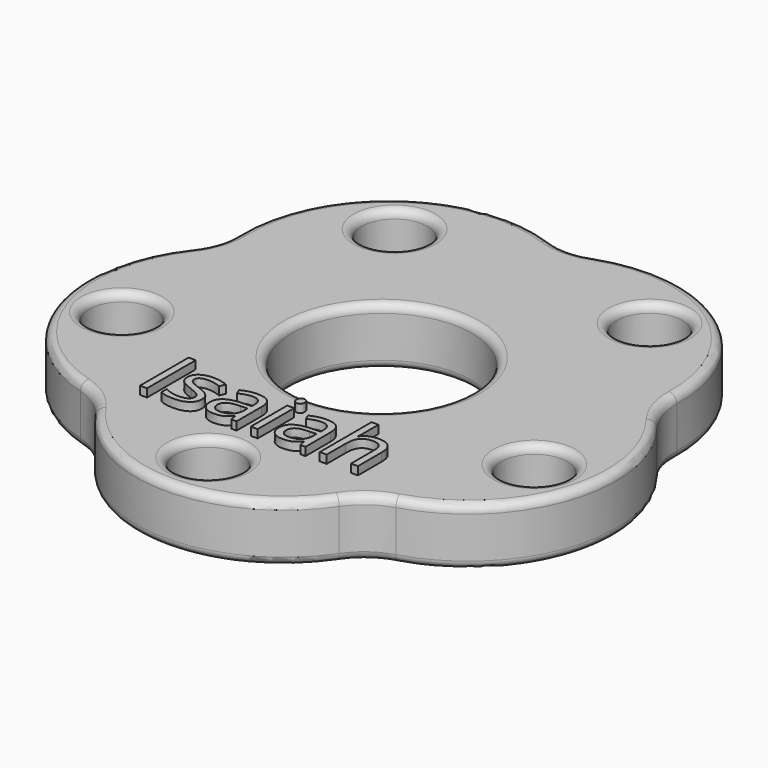
from build123d import *

# Parameters (mm, degrees)
F0_R           = 4
F0_R_2         = 11
F1_DEPTH       = 7.05
F2_R           = 8
F3_R           = 1
F4_TEXT_SIZE   = 10.4166666667
F5_DEPTH       = 1
F6_TEXT_SIZE   = 5.5555555556
F6_TEXT_SIZE_2 = 6.9444444444
F7_DEPTH       = 0.5


# Not quite as in the source:
# - Text() gives the source's letters only with a copy of the font that has no kerning and outlines rounded to 1/6400 em; it was checked with that copy


with BuildPart() as f1:
    # F0 (on Top) → F1 (new body)
    with BuildSketch(Plane.XY):
        with BuildLine():
            ThreePointArc((26.4660662972, 8.5993462218), (19.3969133257, 26.6975608144), (0, 27.8280689357))
            ThreePointArc((0, 27.8280689357), (-19.3969133257, 26.6975608144), (-26.4660662972, 8.5993462218))
            ThreePointArc((-26.4660662972, 8.5993462218), (-31.3848650377, -10.1975608144), (-16.3569285202, -22.5133806896))
            ThreePointArc((-16.3569285202, -22.5133806896), (0, -33), (16.3569285202, -22.5133806896))
            ThreePointArc((16.3569285202, -22.5133806896), (31.3848650377, -10.1975608144), (26.4660662972, 8.5993462218))
        make_face()
        with Locations((0, -26.5)):
            Circle(F0_R, mode=Mode.SUBTRACT)
        with Locations((-25.2029976818, -8.1889503509)):
            Circle(F0_R, mode=Mode.SUBTRACT)
        with Locations((25.2029976818, -8.1889503509)):
            Circle(F0_R, mode=Mode.SUBTRACT)
        Circle(F0_R_2, mode=Mode.SUBTRACT)
        with Locations((-15.5763091858, 21.4389503509)):
            Circle(F0_R, mode=Mode.SUBTRACT)
        with Locations((15.5763091858, 21.4389503509)):
            Circle(F0_R, mode=Mode.SUBTRACT)
    extrude(amount=F1_DEPTH)

    # F2
    f2_edges = [f1.edges().sort_by_distance(p)[0] for p in [
        (16.356929, -22.513381, 3.525),
        (26.466066, 8.599346, 3.525),
        (0, 27.828069, 3.525),
        (-26.466066, 8.599346, 3.525),
        (-16.356929, -22.513381, 3.525),
    ]]
    fillet(f2_edges, radius=F2_R)

    # F3
    f3_edges = [f1.edges().sort_by_distance(p)[0] for p in [
        (0, -33, 7.05),
        (-16.807542, -23.133598, 7.05),
        (16.807542, -23.133598, 7.05),
        (-31.384865, -10.197561, 7.05),
        (31.384865, -10.197561, 7.05),
        (-27.195175, 8.836248, 7.05),
        (27.195175, 8.836248, 7.05),
        (-19.396913, 26.697561, 7.05),
        (19.396913, 26.697561, 7.05),
        (0, 28.594699, 7.05),
        (-4, -26.5, 7.05),
        (-29.202998, -8.18895, 7.05),
        (21.202998, -8.18895, 7.05),
        (-11, 0, 7.05),
        (-19.576309, 21.43895, 7.05),
        (11.576309, 21.43895, 7.05),
        (0, -33, 0),
        (-16.807542, -23.133598, 0),
        (16.807542, -23.133598, 0),
        (-31.384865, -10.197561, 0),
        (31.384865, -10.197561, 0),
        (-27.195175, 8.836248, 0),
        (27.195175, 8.836248, 0),
        (-19.396913, 26.697561, 0),
        (19.396913, 26.697561, 0),
        (0, 28.594699, 0),
        (-4, -26.5, 0),
        (-29.202998, -8.18895, 0),
        (21.202998, -8.18895, 0),
        (-11, 0, 0),
        (-19.576309, 21.43895, 0),
        (11.576309, 21.43895, 0),
    ]]
    fillet(f3_edges, radius=F3_R)

    # F4 (on face) → F5 (join)
    with BuildSketch(Plane.XY.offset(7.05)):
        with Locations((-14.1617838542, -20.5)):
            Text('Isaiah', F4_TEXT_SIZE, font='Open Sans', text_align=(TextAlign.LEFT, TextAlign.BOTTOM))
    extrude(amount=F5_DEPTH)

    # F6 (on face) → F7 (cut)
    with BuildSketch(Plane(origin=(0, 0, 0), x_dir=(1, 0, 0), z_dir=(0, 0, -1))):
        with Locations((-26.6120659722, -2.8942632199)):
            Text('Jesus                  Loves', F6_TEXT_SIZE, font='Open Sans', text_align=(TextAlign.LEFT, TextAlign.BOTTOM))
        with Locations((-7.0643446181, -20.8807812259)):
            Text('You!', F6_TEXT_SIZE_2, font='Open Sans', text_align=(TextAlign.LEFT, TextAlign.BOTTOM))
    extrude(amount=-F7_DEPTH, mode=Mode.SUBTRACT)


solid = f1.part
